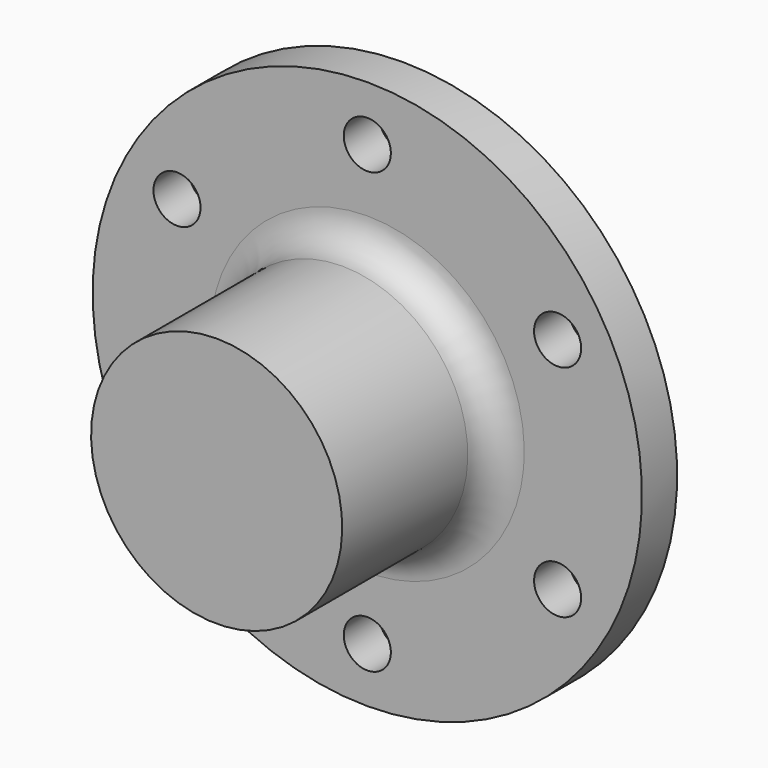
from build123d import *

# Parameters (mm, degrees)
F3_D            = 9.525
F3_COPIES_COUNT = 6


# Not quite as in the source:
# - a pattern or mirror of a feature is missing from the dataset's text; its kind, count and spacing are read off the source's solid


with BuildPart() as f1:
    # F0 (on Right) → F1 (revolve)
    with BuildSketch(Plane.YZ):
        with BuildLine():
            Line((8.89, 55.5625), (0, 55.5625))
            Line((0, 55.5625), (0, 31.75))
            ThreePointArc((0, 31.75), (-1.8598719395, 27.2598719395), (-6.35, 25.4))
            Line((-6.35, 25.4), (-38.1, 25.4))
            Line((-38.1, 25.4), (-38.1, 0))
            Line((-38.1, 0), (-16.51, 0))
            Line((-16.51, 0), (-13.335, 4.7625))
            Line((-13.335, 4.7625), (-9.0805, 4.7625))
            Line((-9.0805, 4.7625), (-3.81, 8.5725))
            Line((-3.81, 8.5725), (-0.7366, 8.5725))
            Line((-0.7366, 8.5725), (7.4295, 13.589))
            Line((7.4295, 13.589), (7.4295, 31.75))
            Line((7.4295, 31.75), (8.89, 31.75))
            Line((8.89, 31.75), (8.89, 55.5625))
        make_face()
    revolve(axis=Axis((0, -27.305, 0), (0, -1, 0)))

    # F3 (through all)
    with Locations(Plane(origin=(0, 8.89, 0), x_dir=(-1, 0, 0), z_dir=(0, 1, 0))):
        with Locations((0, 44.45)):
            f3 = Hole(F3_D / 2)

    # F3_copies: F3 ×6 about axis
    f3_copies_axis = Axis((0, 0, 0), (0, 1, 0))
    for i in range(1, F3_COPIES_COUNT):
        add(f3.rotate(f3_copies_axis, i * 360 / F3_COPIES_COUNT), mode=Mode.SUBTRACT)


solid = f1.part
